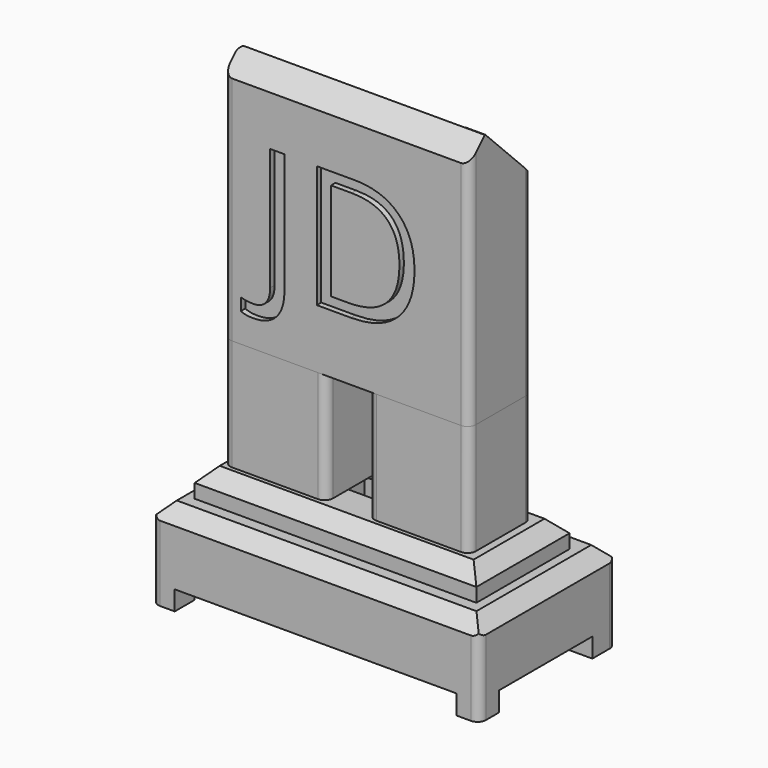
from build123d import *

# Parameters (mm, degrees)
F0_W          = 67.1
F0_H          = 7.1
F1_DEPTH      = 138.3
F2_W          = 88.2
F2_H          = 28.2
F2_W_2        = 74.2
F2_H_2        = 14.2
F3_DEPTH      = 50
F4_W          = 36.8519453004
F4_H          = 28.2
F5_DEPTH      = 40
F4_W_2        = 36.3480546996
F6_W          = 101.2075915933
F6_H          = 41.8235324323
F7_DEPTH      = 10
F8_W          = 18.1213915348
F8_H          = 8.8705555536
F9_DEPTH      = 25
F10_W         = 117.6467612386
F10_H         = 61.5334026515
F10_W_2       = 101.2075915933
F10_H_2       = 41.8235324323
F11_DEPTH     = 25
F12_W         = 7
F12_H         = 21.2
F13_DEPTH     = 40
F14_SIZE      = 21
F15_SIZE      = 7
F16_R         = 3
F17_R         = 3
F18_R         = 3
F18_2_R       = 3
F19_R         = 3
F19_2_R       = 3
F20_R         = 3
F20_2_R       = 3
F21_SIZE      = 5
F22_SIZE      = 5
F23_SIZE      = 5
F24_SIZE      = 5
F25_SIZE      = 5
F26_SIZE      = 5
F27_SIZE      = 5
F28_R         = 3
F28_2_R       = 3
F29_R         = 2
F30_R         = 2
F31_R         = 2
F32_W         = 8.2512535155
F32_H         = 8.9678335935
F32_H_2       = 10.7420366257
F32_W_2       = 8.1879161298
F33_DEPTH     = 7
F34_R         = 3
F36_TEXT_SIZE = 61.5635550477
F37_DEPTH     = 2


# Not quite as in the source:
# - Text() gives the source's letters only with a copy of the font that has no kerning and outlines rounded to 1/6400 em; it was checked with that copy


with BuildPart() as f1:
    # F0 (on Top) → F1 (new body)
    with BuildSketch(Plane.XY):
        with Locations((-0.3188236151, -0.3930132923)):
            Rectangle(F0_W, F0_H)
    extrude(amount=F1_DEPTH)


with BuildPart() as f3:
    # F2 (on Top) → F3 (new body)
    with BuildSketch(Plane.XY):
        with Locations((-0.368696662, -0.4890732596)):
            Rectangle(F2_W, F2_H)
        with Locations((-0.368696662, -0.4890732596)):
            Rectangle(F2_W_2, F2_H_2, mode=Mode.SUBTRACT)
    extrude(amount=F3_DEPTH)

    # F12 (on face) → F13 (join)
    with BuildSketch(Plane.XY.offset(50)):
        Polygon((36.731303338, -7.5890732596), (-44.468696662, -7.5890732596), (-44.468696662, -14.5890732596), (43.731303338, -14.5890732596), (43.731303338, -7.5890732596), align=None)
        with Locations((40.231303338, 3.0109267404)):
            Rectangle(F12_W, F12_H)
    extrude(amount=F13_DEPTH)

    # F14
    f14_edges = [f3.edges().sort_by_distance(p)[0] for p in [
        (40.231303, 13.610927, 90),
    ]]
    chamfer(f14_edges, length=F14_SIZE)

    # F15
    f15_edges = [f3.edges().sort_by_distance(p)[0] for p in [
        (-0.368697, -14.589073, 90),
    ]]
    chamfer(f15_edges, length=F15_SIZE)

    # F16
    f16_edges = [f3.edges().sort_by_distance(p)[0] for p in [
        (-44.468697, 13.610927, 25),
    ]]
    fillet(f16_edges, radius=F16_R)

    # F17
    f17_edges = [f3.edges().sort_by_distance(p)[0] for p in [
        (43.731303, 13.610927, 34.5),
    ]]
    fillet(f17_edges, radius=F17_R)

    # F19
    f19_edges = [f3.edges().sort_by_distance(p)[0] for p in [
        (43.731303, -14.589073, 41.5),
    ]]
    fillet(f19_edges, radius=F19_R)

    # F20
    f20_edges = [f3.edges().sort_by_distance(p)[0] for p in [
        (-44.468697, -14.589073, 41.5),
    ]]
    fillet(f20_edges, radius=F20_R)

    # F29
    f29_edges = [f3.edges().sort_by_distance(p)[0] for p in [
        (-2.368697, 13.610927, 50),
    ]]
    fillet(f29_edges, radius=F29_R)

    # F30
    f30_edges = [f3.edges().sort_by_distance(p)[0] for p in [
        (-44.468697, -7.589073, 70),
    ]]
    fillet(f30_edges, radius=F30_R)

    # F31
    f31_edges = [f3.edges().sort_by_distance(p)[0] for p in [
        (36.731303, 13.610927, 59.5),
    ]]
    fillet(f31_edges, radius=F31_R)

    # F36 (on face) → F37 (cut)
    with BuildSketch(Plane.XZ.offset(14.5890732596)):
        with Locations((-33.5190668702, 21.2174449116)):
            Text('JD', F36_TEXT_SIZE, font='Open Sans', text_align=(TextAlign.LEFT, TextAlign.BOTTOM))
    extrude(amount=-F37_DEPTH, mode=Mode.SUBTRACT)


with BuildPart() as f5:
    # F4 (on face) → F5 (new body)
    with BuildSketch(Plane(origin=(0, 0, 0), x_dir=(1, 0, 0), z_dir=(0, 0, -1))):
        with Locations((-26.0427240118, 0.4890732596)):
            Rectangle(F4_W, F4_H)
    extrude(amount=F5_DEPTH)

    # F18
    f18_edges = [f5.edges().sort_by_distance(p)[0] for p in [
        (-44.468697, 13.610927, -20),
    ]]
    fillet(f18_edges, radius=F18_R)

    # F20#2
    f20_2_edges = [f5.edges().sort_by_distance(p)[0] for p in [
        (-44.468697, -14.589073, -20),
    ]]
    fillet(f20_2_edges, radius=F20_2_R)

    # F28
    f28_edges = [f5.edges().sort_by_distance(p)[0] for p in [
        (-7.616751, 13.610927, -20),
        (-7.616751, -14.589073, -20),
    ]]
    fillet(f28_edges, radius=F28_R)


with BuildPart() as f5b:
    # F4 (on face) → F5, piece 2 (new body)
    with BuildSketch(Plane(origin=(0, 0, 0), x_dir=(1, 0, 0), z_dir=(0, 0, -1))):
        with Locations((25.5572759882, 0.4890732596)):
            Rectangle(F4_W_2, F4_H)
    extrude(amount=F5_DEPTH)

    # F18#2
    f18_2_edges = [f5b.edges().sort_by_distance(p)[0] for p in [
        (43.731303, 13.610927, -20),
    ]]
    fillet(f18_2_edges, radius=F18_2_R)

    # F19#2
    f19_2_edges = [f5b.edges().sort_by_distance(p)[0] for p in [
        (43.731303, -14.589073, -20),
    ]]
    fillet(f19_2_edges, radius=F19_2_R)

    # F28#2
    f28_2_edges = [f5b.edges().sort_by_distance(p)[0] for p in [
        (7.383249, -14.589073, -20),
        (7.383249, 13.610927, -20),
    ]]
    fillet(f28_2_edges, radius=F28_2_R)


with BuildPart() as f7:
    # F6 (on face) → F7 (new body)
    with BuildSketch(Plane(origin=(0, 0, -40), x_dir=(1, 0, 0), z_dir=(0, 0, -1))):
        with Locations((0.8287318051, 0.0900365412)):
            Rectangle(F6_W, F6_H)
    extrude(amount=F7_DEPTH)

    # F8 (on face) → F9 (cut)
    with BuildSketch(Plane(origin=(0, 0, -50), x_dir=(1, 0, 0), z_dir=(0, 0, -1))):
        with Locations((0.1267595217, 0.251886202)):
            Rectangle(F8_W, F8_H)
    extrude(amount=-F9_DEPTH, mode=Mode.SUBTRACT)

    # F21
    f21_edges = [f7.edges().sort_by_distance(p)[0] for p in [
        (0.828732, 20.82173, -40),
    ]]
    chamfer(f21_edges, length=F21_SIZE)

    # F22
    f22_edges = [f7.edges().sort_by_distance(p)[0] for p in [
        (-49.775064, -2.590037, -40),
    ]]
    chamfer(f22_edges, length=F22_SIZE)

    # F23
    f23_edges = [f7.edges().sort_by_distance(p)[0] for p in [
        (51.432528, -2.590037, -40),
    ]]
    chamfer(f23_edges, length=F23_SIZE)

    # F24
    f24_edges = [f7.edges().sort_by_distance(p)[0] for p in [
        (0.828732, -21.001803, -40),
    ]]
    chamfer(f24_edges, length=F24_SIZE)


with BuildPart() as f11:
    # F10 (on face) → F11 (new body)
    with BuildSketch(Plane(origin=(0, 0, -50), x_dir=(1, 0, 0), z_dir=(0, 0, -1))):
        with Locations((0.7970631123, -0.7970649749)):
            Rectangle(F10_W, F10_H)
        with Locations((0.8287318051, 0.0900365412)):
            Rectangle(F10_W_2, F10_H_2, mode=Mode.SUBTRACT)
    extrude(amount=F11_DEPTH)

    # F25
    f25_edges = [f11.edges().sort_by_distance(p)[0] for p in [
        (0.797063, 31.563766, -50),
    ]]
    chamfer(f25_edges, length=F25_SIZE)

    # F26
    f26_edges = [f11.edges().sort_by_distance(p)[0] for p in [
        (59.620444, -1.702935, -50),
        (0.797063, -29.969636, -50),
    ]]
    chamfer(f26_edges, length=F26_SIZE)

    # F27
    f27_edges = [f11.edges().sort_by_distance(p)[0] for p in [
        (-58.026318, 0.797065, -50),
    ]]
    chamfer(f27_edges, length=F27_SIZE)

    # F32 (on face) → F33 (join)
    with BuildSketch(Plane(origin=(0, 0, -75), x_dir=(1, 0, 0), z_dir=(0, 0, -1))):
        with Locations((-53.9006907493, 25.4857195541)):
            Rectangle(F32_W, F32_H)
        with Locations((-53.9006907493, -26.1927479878)):
            Rectangle(F32_W, F32_H_2)
        with Locations((55.5264856666, 25.4857195541)):
            Rectangle(F32_W_2, F32_H)
        with Locations((55.5264856666, -26.1927479878)):
            Rectangle(F32_W_2, F32_H_2)
    extrude(amount=F33_DEPTH)

    # F34
    f34_edges = [f11.edges().sort_by_distance(p)[0] for p in [
        (-58.026318, 31.563766, -68.5),
        (-58.026318, -29.969636, -68.5),
        (59.620444, 31.563766, -68.5),
        (59.620444, -29.969636, -68.5),
    ]]
    fillet(f34_edges, radius=F34_R)


solid = Compound([f3.part, f5.part, f5b.part, f7.part, f11.part])
